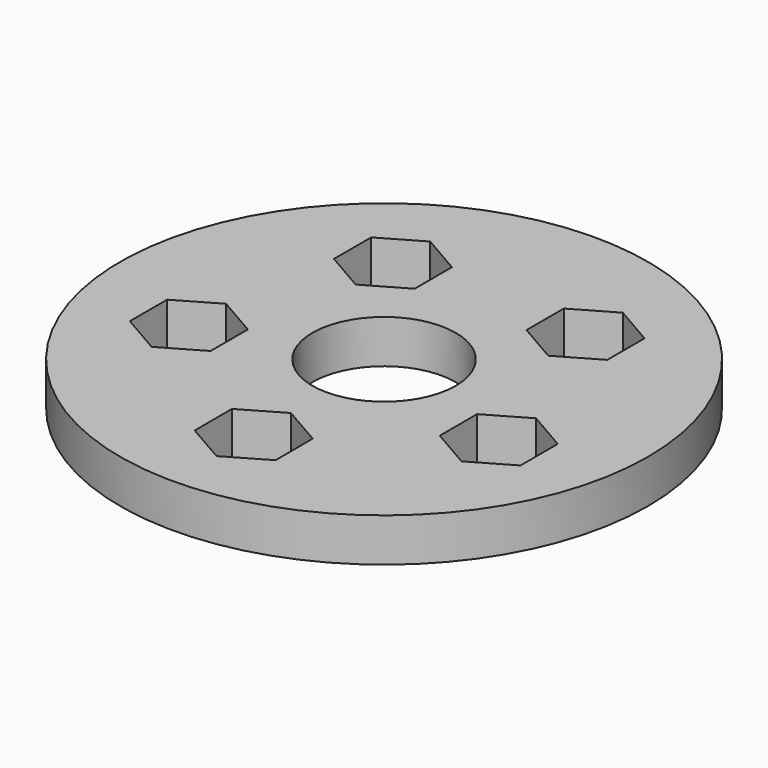
from build123d import *

# Parameters (mm, degrees)
F0_R     = 40.5
F1_DEPTH = 6.66


# Not quite as in the source:
# - a feature names something its author has since deleted; it is built from what else it names


with BuildPart() as f1:
    # F0 (on Top) → F1 (new body)
    with BuildSketch(Plane.XY):
        Circle(F0_R)
        Polygon((-23.7764129074, -14.8754248594), (-29.9684945444, -11.3004248594), (-29.9684945444, -4.1504248594), (-23.7764129074, -0.5754248594), (-17.5843312703, -4.1504248594), (-17.5843312703, -11.3004248594), align=None, mode=Mode.SUBTRACT)
        Polygon((-0.0180177662, -17.8500227021), (0, -17.8603648131), (6.1830530933, -21.4094075078), (6.2010708595, -28.5593848057), (0.0180177662, -32.1499772979), (-6.1830530933, -28.5905924922), (-6.2010708595, -21.4406151943), align=None, mode=Mode.SUBTRACT)
        Polygon((23.7764129074, -0.5754248594), (29.9684945444, -4.1504248594), (29.9684945444, -11.3004248594), (23.7764129074, -14.8754248594), (17.5843312703, -11.3004248594), (17.5843312703, -4.1504248594), align=None, mode=Mode.SUBTRACT)
        Polygon((-14.7765176587, 27.3156769259), (-8.5844360217, 23.7406769259), (-8.5844360217, 16.5906769259), (-14.7765176587, 13.0156769259), (-20.9685992958, 16.5906769259), (-20.9685992958, 23.7406769259), align=None, mode=Mode.SUBTRACT)
        with BuildLine():
            ThreePointArc((0, -11), (-7.7781745931, 7.7781745931), (11, 0))
            ThreePointArc((11, 0), (7.7781745931, -7.7781745931), (0, -11))
        make_face(mode=Mode.SUBTRACT)
        Polygon((14.7765176587, 27.3156769259), (20.9685992958, 23.7406769259), (20.9685992958, 16.5906769259), (14.7765176587, 13.0156769259), (8.5844360217, 16.5906769259), (8.5844360217, 23.7406769259), align=None, mode=Mode.SUBTRACT)
    extrude(amount=F1_DEPTH)


solid = f1.part
